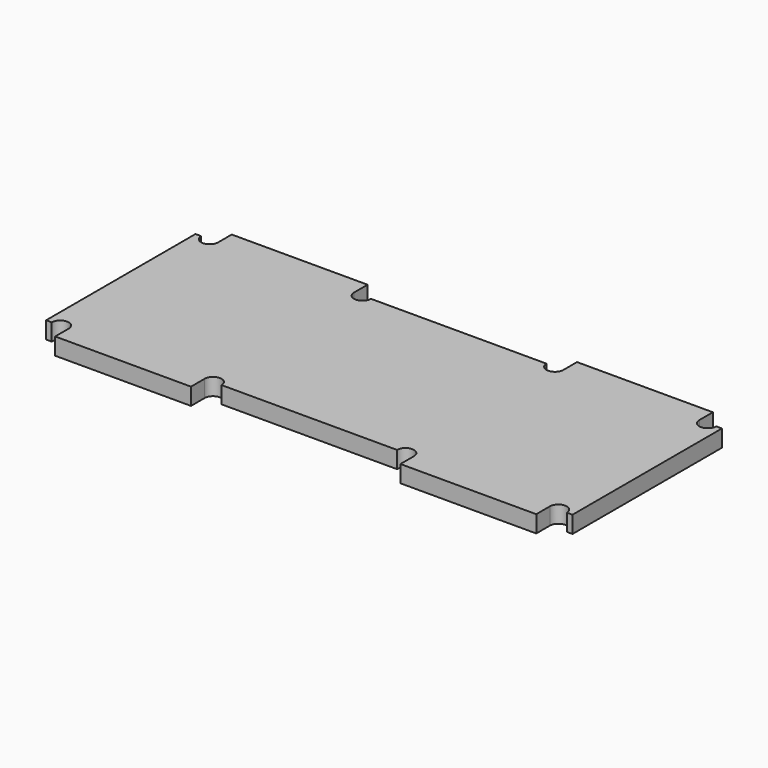
from build123d import *

# Parameters (mm, degrees)
F1_W     = 590.55
F1_H     = 209.55
F2_DEPTH = 19.05
F3_W     = 152.4
F3_H     = 247.65
F4_DEPTH = 19.05
F6_DEPTH = 25.4


# Not quite as in the source:
# - a variable given as a bare number and used for a length is read in inches; the dataset says mm whatever the document's units were


with BuildPart() as f2:
    # F1 (on Top) → F2 (new body)
    with BuildSketch(Plane.XY):
        Rectangle(F1_W, F1_H)
    extrude(amount=F2_DEPTH)

    # F3 (on face) → F4 (join)
    with BuildSketch(Plane.XY.offset(19.05)):
        with Locations((-193.675, 0)):
            Rectangle(F3_W, F3_H)
        with Locations((193.675, 0)):
            Rectangle(F3_W, F3_H)
    extrude(amount=-F4_DEPTH)

    # F5 (on face) → F6 (cut)
    with BuildSketch(Plane.XY.offset(19.05)):
        with BuildLine():
            Line((-98.425, 104.775), (-117.475, 104.775))
            ThreePointArc((-117.475, 104.775), (-107.95, 95.25), (-98.425, 104.775))
        make_face()
        with BuildLine():
            ThreePointArc((-98.425, 104.775), (-107.95, 114.3), (-117.475, 104.775))
            Line((-117.475, 104.775), (-98.425, 104.775))
        make_face()
        with BuildLine():
            Line((-117.475, -104.775), (-98.425, -104.775))
            ThreePointArc((-98.425, -104.775), (-107.95, -95.25), (-117.475, -104.775))
        make_face()
        with BuildLine():
            Line((98.425, -104.775), (117.475, -104.775))
            ThreePointArc((117.475, -104.775), (107.95, -95.25), (98.425, -104.775))
        make_face()
        with BuildLine():
            Line((117.475, 104.775), (98.425, 104.775))
            ThreePointArc((98.425, 104.775), (107.95, 95.25), (117.475, 104.775))
        make_face()
        with BuildLine():
            Line((288.925, 104.775), (269.875, 104.775))
            ThreePointArc((269.875, 104.775), (279.4, 95.25), (288.925, 104.775))
        make_face()
        with BuildLine():
            Line((269.875, -104.775), (288.925, -104.775))
            ThreePointArc((288.925, -104.775), (279.4, -95.25), (269.875, -104.775))
        make_face()
        with BuildLine():
            Line((-288.925, -104.775), (-269.875, -104.775))
            ThreePointArc((-269.875, -104.775), (-279.4, -95.25), (-288.925, -104.775))
        make_face()
        with BuildLine():
            Line((-269.875, 104.775), (-288.925, 104.775))
            ThreePointArc((-288.925, 104.775), (-279.4, 95.25), (-269.875, 104.775))
        make_face()
    extrude(amount=-F6_DEPTH, mode=Mode.SUBTRACT)


solid = f2.part
